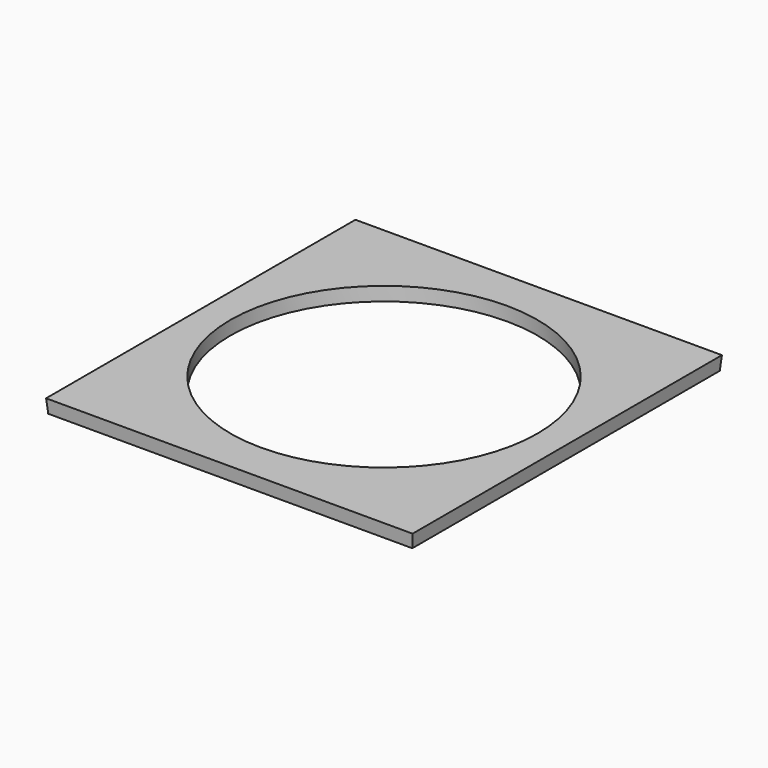
from build123d import *

# Parameters (mm, degrees)
F0_W         = 79.5695781708
F0_H         = 83.9737951756
F1_DEPTH     = 3
F1_TAPER     = -5
F2_R         = 33.5765406983
F3_DEPTH     = 80
F4_TEXT_SIZE = 10.7193495043
F5_DEPTH     = 5


# Not quite as in the source:
# - Text() gives the source's letters only with a copy of the font that has no kerning and outlines rounded to 1/6400 em; it was checked with that copy


with BuildPart() as f1:
    # F0 (on Top) → F1 (new body)
    with BuildSketch(Plane.XY):
        Rectangle(F0_W, F0_H)
    extrude(amount=F1_DEPTH, taper=F1_TAPER)

    # F2 (on face) → F3 (cut)
    with BuildSketch(Plane.XY.offset(3)):
        Circle(F2_R)
    extrude(amount=-F3_DEPTH, mode=Mode.SUBTRACT)

    # F4 (on face) → F5 (cut)
    with BuildSketch(Plane(origin=(0, -41.6679599286, -3.645474126), x_dir=(1, 0, 0), z_dir=(0, -0.9961946981, -0.0871557427))):
        with Locations((-37.5579208258, 22.261813283)):
            Text('Leothek', F4_TEXT_SIZE, font='Open Sans', font_style=FontStyle.ITALIC, text_align=(TextAlign.LEFT, TextAlign.BOTTOM))
    extrude(amount=-F5_DEPTH, mode=Mode.SUBTRACT)


solid = f1.part
